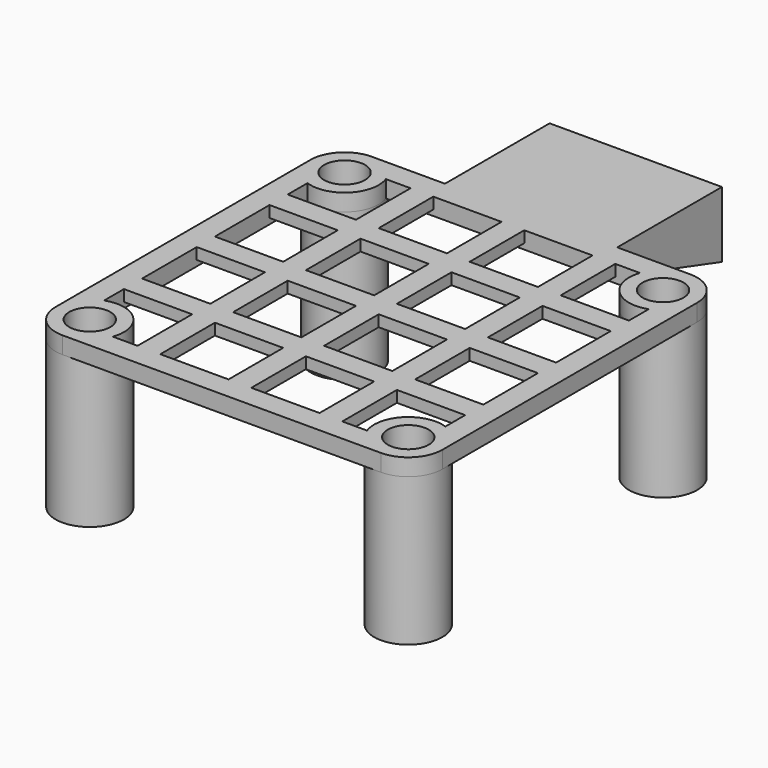
from build123d import *
from build123d import SkipClean  # not in build123d's __all__

# Parameters (mm, degrees)
F0_R      = 3
F0_R_2    = 1.8
F1_DEPTH  = 13
F2_R      = 1.8
F3_DEPTH  = 1.5
F4_W      = 6
F4_H      = 6
F5_DEPTH  = 1
F6_W      = 15.15
F6_H      = 11.5
F7_DEPTH  = 5.8
F8_W      = 12.75
F8_H      = 7
F9_DEPTH  = 4.6
F10_W     = 11.75
F10_H     = 3.56
F11_DEPTH = 4
F13_DEPTH = 2
F15_DEPTH = 25


with BuildPart() as f1:
    # F0 (on Top) → F1 (new body)
    with BuildSketch(Plane.XY):
        with Locations((-14, 14)):
            Circle(F0_R)
        with Locations((-14, 14)):
            Circle(F0_R_2, mode=Mode.SUBTRACT)
    extrude(amount=F1_DEPTH)



with BuildPart() as f1b:
    # F0 (on Top) → F1, piece 2 (new body)
    with BuildSketch(Plane.XY):
        with Locations((-14, -14)):
            Circle(F0_R)
        with Locations((-14, -14)):
            Circle(F0_R_2, mode=Mode.SUBTRACT)
    extrude(amount=F1_DEPTH)


with BuildPart() as f1c:
    # F0 (on Top) → F1, piece 3 (new body)
    with BuildSketch(Plane.XY):
        with Locations((14, -14)):
            Circle(F0_R)
        with Locations((14, -14)):
            Circle(F0_R_2, mode=Mode.SUBTRACT)
    extrude(amount=F1_DEPTH)


with BuildPart() as f1d:
    # F0 (on Top) → F1, piece 4 (new body)
    with BuildSketch(Plane.XY):
        with Locations((14, 14)):
            Circle(F0_R)
        with Locations((14, 14)):
            Circle(F0_R_2, mode=Mode.SUBTRACT)
    extrude(amount=F1_DEPTH)


with BuildPart() as f1_1:
    add(f1.part, clean=False)

    with SkipClean():  # cleaning this boolean's faces spoils the solid; the shape is the same uncleaned
        add(f1b.part)  # F3 merges F1b

    with SkipClean():  # cleaning this boolean's faces spoils the solid; the shape is the same uncleaned
        add(f1c.part)  # F3 merges F1c

    with SkipClean():  # cleaning this boolean's faces spoils the solid; the shape is the same uncleaned
        add(f1d.part)  # F3 merges F1d
    # F2 (on face) → F3 (join)
    with BuildSketch(Plane.XY.offset(13)):
        with BuildLine():
            Line((14, 17), (-14, 17))
            ThreePointArc((-14, 17), (-16.1213203436, 16.1213203436), (-17, 14))
            Line((-17, 14), (-17, -14))
            ThreePointArc((-17, -14), (-16.1213203436, -16.1213203436), (-14, -17))
            Line((-14, -17), (14, -17))
            ThreePointArc((14, -17), (16.1213203436, -16.1213203436), (17, -14))
            Line((17, -14), (17, 14))
            ThreePointArc((17, 14), (16.1213203436, 16.1213203436), (14, 17))
        make_face()
        with Locations((-14, -14)):
            Circle(F2_R, mode=Mode.SUBTRACT)
        with Locations((14, -14)):
            Circle(F2_R, mode=Mode.SUBTRACT)
        with Locations((-14, 14)):
            Circle(F2_R, mode=Mode.SUBTRACT)
        with BuildLine():
            Line((-15, -11.1715728753), (-15, 11.1715728753))
            ThreePointArc((-15, 11.1715728753), (-11.8786796564, 11.8786796564), (-11.1715728753, 15))
            Line((-11.1715728753, 15), (11.1715728753, 15))
            ThreePointArc((11.1715728753, 15), (11.8786796564, 11.8786796564), (15, 11.1715728753))
            Line((15, 11.1715728753), (15, -11.1715728753))
            ThreePointArc((15, -11.1715728753), (11.8786796564, -11.8786796564), (11.1715728753, -15))
            Line((11.1715728753, -15), (-11.1715728753, -15))
            ThreePointArc((-11.1715728753, -15), (-11.8786796564, -11.8786796564), (-15, -11.1715728753))
        make_face(mode=Mode.SUBTRACT)
        with Locations((14, 14)):
            Circle(F2_R, mode=Mode.SUBTRACT)
    with SkipClean():  # cleaning this boolean's faces spoils the solid; the shape is the same uncleaned
        extrude(amount=F3_DEPTH)

    # F4 (on face) → F5 (join)
    with BuildSketch(Plane.XY.offset(14.5)):
        Polygon((1, 15), (-1, 15), (-1, 9), (-7, 9), (-7, 15), (-9, 15), (-9, 9), (-15, 9), (-15, 7), (-9, 7), (-9, 1), (-15, 1), (-15, -1), (-9, -1), (-9, -7), (-15, -7), (-15, -9), (-9, -9), (-9, -15), (-7, -15), (-7, -9), (-1, -9), (-1, -15), (1, -15), (1, -9), (7, -9), (7, -15), (9, -15), (9, -9), (15, -9), (15, -7), (9, -7), (9, -1), (15, -1), (15, 1), (9, 1), (9, 7), (15, 7), (15, 9), (9, 9), (9, 15), (7, 15), (7, 9), (1, 9), align=None)
        with Locations((-4, -4)):
            Rectangle(F4_W, F4_H, mode=Mode.SUBTRACT)
        with Locations((4, -4)):
            Rectangle(F4_W, F4_H, mode=Mode.SUBTRACT)
        with Locations((-4, 4)):
            Rectangle(F4_W, F4_H, mode=Mode.SUBTRACT)
        with Locations((4, 4)):
            Rectangle(F4_W, F4_H, mode=Mode.SUBTRACT)
    extrude(amount=-F5_DEPTH)

    # F6 (on face) → F7 (join)
    with BuildSketch(Plane.XY.offset(14.5)):
        with Locations((0, 22.75)):
            Rectangle(F6_W, F6_H)
    with SkipClean():  # cleaning this boolean's faces spoils the solid; the shape is the same uncleaned
        extrude(amount=-F7_DEPTH)

    # F8 (on face) → F9 (cut)
    with BuildSketch(Plane(origin=(0, 0, 8.7), x_dir=(1, 0, 0), z_dir=(0, 0, -1))):
        with Locations((0, -20.5)):
            Rectangle(F8_W, F8_H)
    with SkipClean():  # cleaning this boolean's faces spoils the solid; the shape is the same uncleaned
        extrude(amount=-F9_DEPTH, mode=Mode.SUBTRACT)

    # F10 (on face) → F11 (cut)
    with BuildSketch(Plane(origin=(0, 0, 8.7), x_dir=(1, 0, 0), z_dir=(0, 0, -1))):
        with Locations((0, -25.78)):
            Rectangle(F10_W, F10_H)
    with SkipClean():  # cleaning this boolean's faces spoils the solid; the shape is the same uncleaned
        extrude(amount=-F11_DEPTH, mode=Mode.SUBTRACT)

    # F12 (on face) → F13 (cut, symmetric)
    with BuildSketch(Plane(origin=(0, 28.5, 0), x_dir=(-1, 0, 0), z_dir=(0, 1, 0))):
        with BuildLine():
            Line((-4, 8.7), (4, 8.7))
            ThreePointArc((4, 8.7), (0, 12.7), (-4, 8.7))
        make_face()
    with SkipClean():  # cleaning this boolean's faces spoils the solid; the shape is the same uncleaned
        extrude(amount=F13_DEPTH, both=True, mode=Mode.SUBTRACT)

    # F14 (on face) → F15 (cut)
    with BuildSketch(Plane(origin=(-7.575, 0, 0), x_dir=(0, -1, 0), z_dir=(-1, 0, 0))):
        Polygon((-17, 12.2429373081), (-28.5, 8.7), (-17, 8.7), align=None)
    extrude(amount=-F15_DEPTH, mode=Mode.SUBTRACT)


solid = f1_1.part
